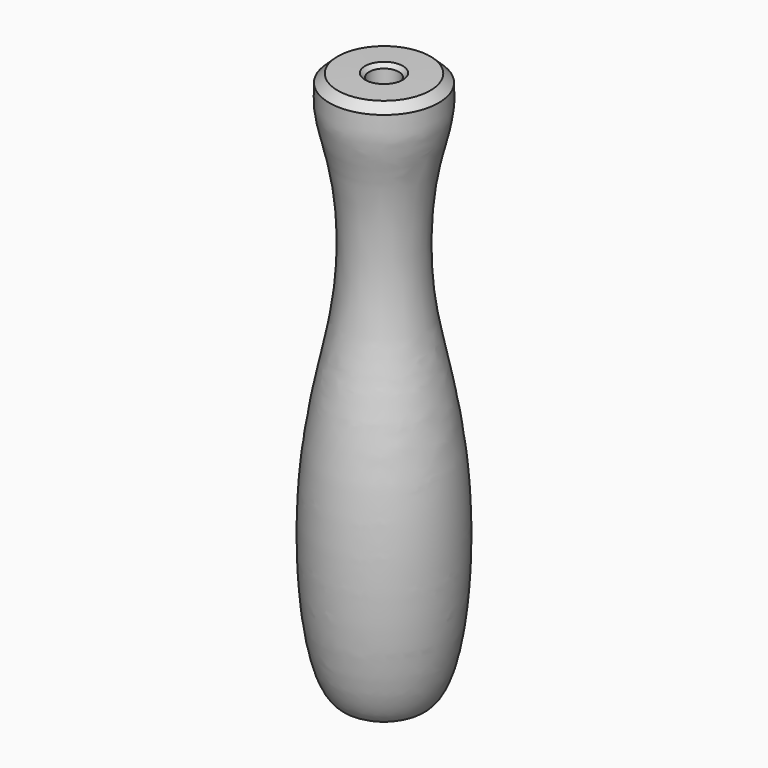
from build123d import *

# Parameters (mm, degrees)
F2_SIZE = 0.5


# Not quite as in the source:
# - a fillet or chamfer that OpenCascade refuses, or shapes differently, is made with other operations: its cross-section is extruded or revolved along the edge and cut away or added


with BuildPart() as f1:
    # F0 (on Front) → F1 (revolve)
    with BuildSketch(Plane.XZ):
        with BuildLine():
            Line((0, -70), (0, -38))
            Line((0, -38), (-1.285, -38))
            Line((-1.285, -38), (-1.9, 0))
            Line((-1.9, 0), (-6.8993453069, -0.0809104569))
            add(Edge.make_bspline(
                [(-6.8993453069, -0.0809104569), (-7.0014603061, -1.4440725122), (-7.2371386125, -4.5902089989), (-4.8192908443, -11.5999377193), (-4.3986237704, -23.9254930043), (-7.1827283169, -34.8345330377), (-9.5576079288, -50.1893109589), (-7.3330742685, -72.3630189234), (-1.871357568, -70.6030285776), (0, -70)],
                knots=[0, 0, 0, 0, 0.0924718936, 0.2134223127, 0.3696075366, 0.5186517332, 0.7036837237, 0.8984726348, 1, 1, 1, 1], degree=3))
        make_face()
    revolve(axis=Axis((0, 0, -54), (0, 0, 1)))

    # F2
    f2_edges = [f1.edges().sort_by_distance(p)[0] for p in [
        (1.9, 0, 0),
    ]]
    chamfer(f2_edges, length=F2_SIZE)

    # F3: chamfer of 1 on 1 edges, made by hand

    # F3_s1 → F3_t2 (revolve, cut)
    with BuildSketch(Plane.XZ):
        with BuildLine():
            Line((-5.8658675874, -0.0370040548), (-6.9992956914, -1.1211002402))
            Line((-6.9992956914, -1.1211002402), (-7.0192588963, -1.1198876194))
            ThreePointArc((-7.0192588963, -1.1198876194), (-6.9576592361, -0.6004122497), (-6.9192894263, -0.0794164352))
            Line((-6.9192894263, -0.0794164352), (-6.8996689488, -0.0609130757))
            ThreePointArc((-6.8996689488, -0.0609130757), (-6.3827102001, -0.0525465065), (-5.8661912292, -0.0170066736))
            Line((-5.8661912292, -0.0170066736), (-5.8658675874, -0.0370040548))
        make_face()
    revolve(axis=Axis((0, 0, -0.0809104569), (0, 0, 1)), mode=Mode.SUBTRACT)


solid = f1.part
